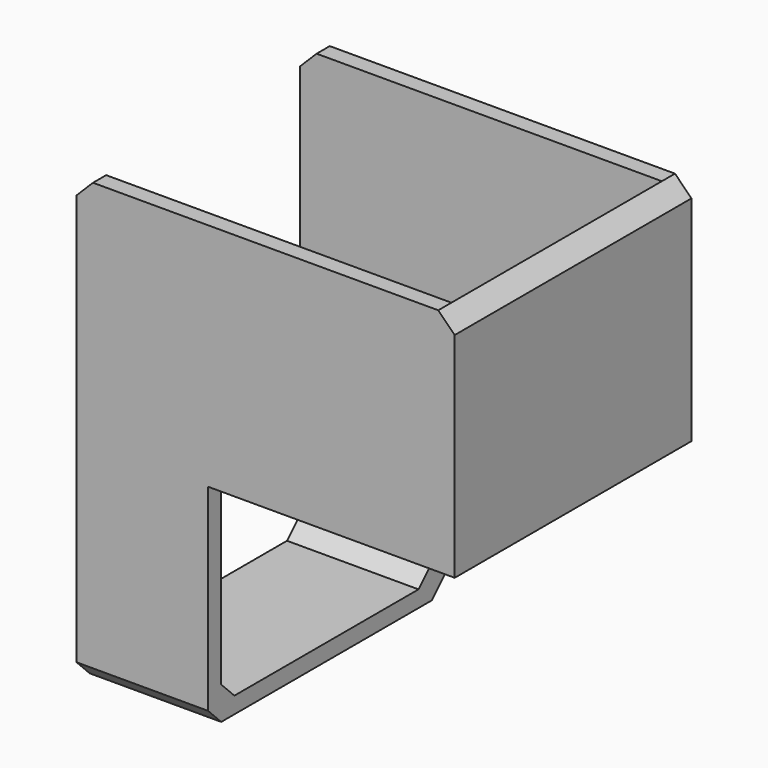
from build123d import *

# Parameters (mm, degrees)
F0_W     = 90
F0_H     = 70
F1_DEPTH = 5
F2_W     = 5
F2_H     = 70
F3_DEPTH = 110
F4_W     = 40
F4_H     = 5
F5_DEPTH = 65
F6_W     = 40
F6_H     = 5
F7_DEPTH = 80
F8_SIZE  = 4.99999


# Not quite as in the source:
# - a fillet or chamfer is up to 0.001 mm smaller than in the source, because OpenCascade refuses the exact size


with BuildPart() as f1:
    # F0 (on Right) → F1 (new body)
    with BuildSketch(Plane.YZ):
        Rectangle(F0_W, F0_H)
    extrude(amount=-F1_DEPTH)

    # F2 (on face) → F3 (join)
    with BuildSketch(Plane(origin=(-5, 0, 0), x_dir=(0, -1, 0), z_dir=(-1, 0, 0))):
        with Locations((-42.5, 0)):
            Rectangle(F2_W, F2_H)
        with Locations((42.5, 0)):
            Rectangle(F2_W, F2_H)
    extrude(amount=F3_DEPTH)

    # F4 (on face) → F5 (join)
    with BuildSketch(Plane(origin=(0, 0, -35), x_dir=(1, 0, 0), z_dir=(0, 0, -1))):
        with Locations((-95, 42.5)):
            Rectangle(F4_W, F4_H)
        with Locations((-95, -42.5)):
            Rectangle(F4_W, F4_H)
    extrude(amount=F5_DEPTH)

    # F6 (on face) → F7 (join, through all)
    with BuildSketch(Plane(origin=(0, -40, 0), x_dir=(-1, 0, 0), z_dir=(0, 1, 0))):
        with Locations((95, -97.5)):
            Rectangle(F6_W, F6_H)
    extrude(amount=F7_DEPTH)

    # F8 (size 5 in the source; OpenCascade refuses exactly that, so slightly less here)
    f8_edges = [f1.edges().sort_by_distance(p)[0] for p in [
        (0, 0, 35),
        (-115, 42.5, 35),
        (-115, -42.5, 35),
        (-95, -45, -100),
        (-95, -40, -95),
        (-95, 40, -95),
        (-95, 45, -100),
    ]]
    chamfer(f8_edges, length=F8_SIZE)


solid = f1.part
